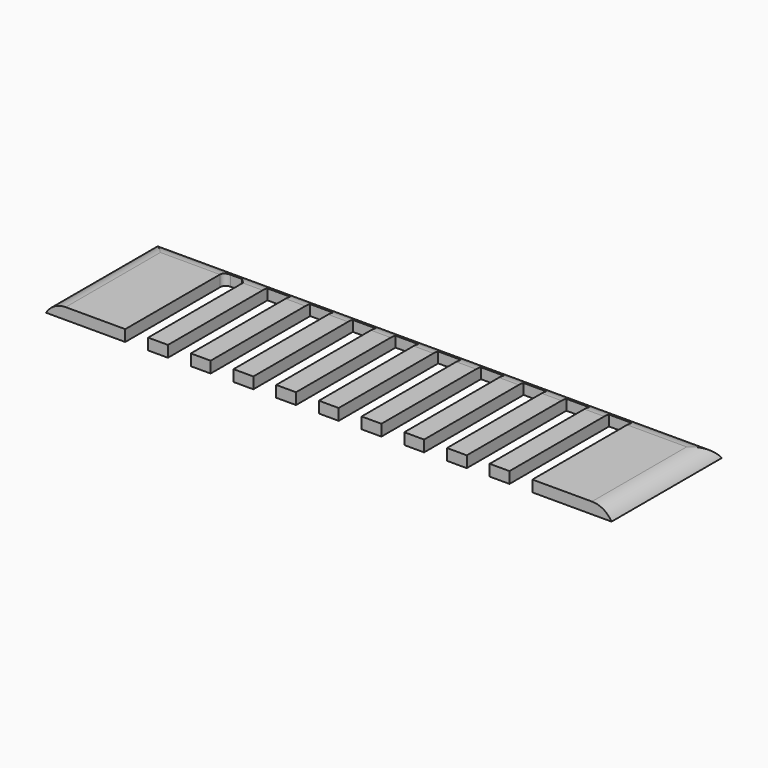
from build123d import *

# Parameters (mm, degrees)
F1_DEPTH    = 2
F2_T1_DEPTH = 67.3205080757
F3_T1_DEPTH = 38.2564064606
F5_R        = 1
F6_SIZE     = 1


# Not quite as in the source:
# - a fillet or chamfer that OpenCascade refuses, or shapes differently, is made with other operations: its cross-section is extruded or revolved along the edge and cut away or added


with BuildPart() as f1:
    # F0 (on Top) → F1 (new body)
    with BuildSketch(Plane.XY):
        Polygon((-1.75, 0), (0, 0), (0, 24.4), (-50, 24.4), (-50, 0), (-36, 0), (-36, 22), (-31.95, 22), (-31.95, 0), (-28.45, 0), (-28.45, 22), (-24.4, 22), (-24.4, 0), (-20.9, 0), (-20.9, 22), (-16.85, 22), (-16.85, 0), (-13.35, 0), (-13.35, 22), (-9.3, 22), (-9.3, 0), (-5.8, 0), (-5.8, 22), (-1.75, 22), align=None)
    extrude(amount=F1_DEPTH)

    # F2: fillet of radius 4 on 1 edges, made by hand

    # F2_s2 → F2_t1 (cut)
    with BuildSketch(Plane.YZ.offset(-58.6602540378)):
        with BuildLine():
            ThreePointArc((24.4, 0), (22.9358983849, 1.4641016151), (20.9358983849, 2))
            Line((20.9358983849, 2), (24.4, 2))
            Line((24.4, 2), (24.4, 0))
        make_face()
    extrude(amount=F2_T1_DEPTH, mode=Mode.SUBTRACT)

    # F3: fillet of radius 4 on 1 edges, made by hand

    # F3_s2 → F3_t1 (cut)
    with BuildSketch(Plane.XZ.offset(-29.5961524227)):
        with BuildLine():
            ThreePointArc((-50, 0), (-48.5358983849, 1.4641016151), (-46.5358983849, 2))
            Line((-46.5358983849, 2), (-50, 2))
            Line((-50, 2), (-50, 0))
        make_face()
    extrude(amount=F3_T1_DEPTH, mode=Mode.SUBTRACT)

    # F4: F1 across plane


with BuildPart() as f1_1:
    add(f1.part)
    add(f1.part.mirror(Plane.YZ))

    # F5
    f5_edges = [f1_1.edges().sort_by_distance(p)[0] for p in [
        (-36, 22, 0.927932),
    ]]
    fillet(f5_edges, radius=F5_R)

    # F6
    f6_edges = [f1_1.edges().sort_by_distance(p)[0] for p in [
        (-31.95, 22, 0.927932),
    ]]
    chamfer(f6_edges, length=F6_SIZE)


solid = f1_1.part
